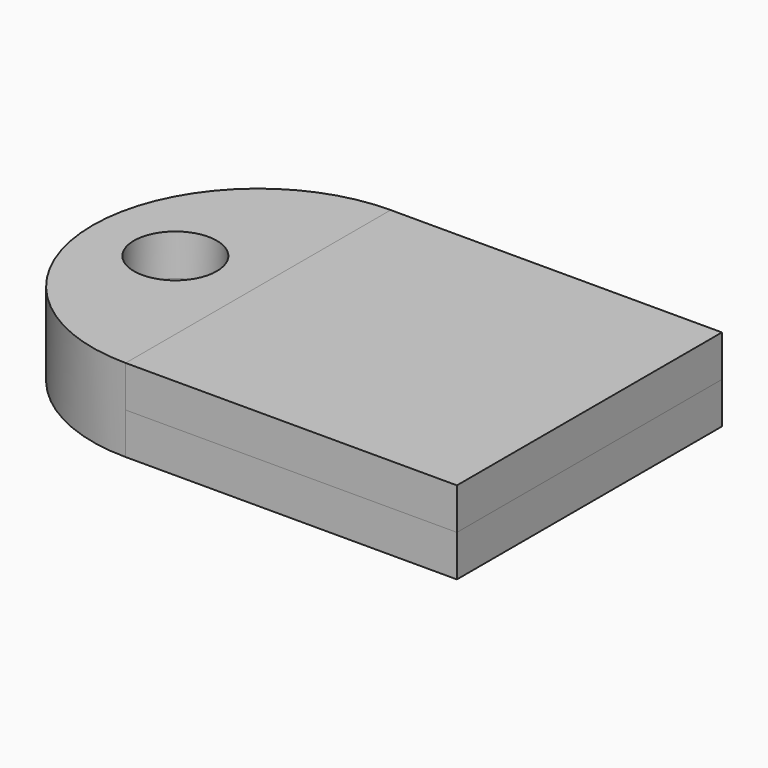
from build123d import *

# Parameters (mm, degrees)
F0_R          = 6.35
F1_DEPTH      = 6.35
F1_DEPTH_BACK = 6.35
F0_W          = 50.8
F0_H          = 50.8
F2_DEPTH      = 6.35
F3_DEPTH      = 6.35
F4_DEPTH      = 6.35


with BuildPart() as f1:
    # F0 (on Top) → F1 (new body, two sides)
    with BuildSketch(Plane.XY) as f1_sk:
        with BuildLine():
            Line((-25.4, -25.4), (-25.4, 25.4))
            ThreePointArc((-25.4, 25.4), (-50.8, 0), (-25.4, -25.4))
        make_face()
        with Locations((-38.1, 0)):
            Circle(F0_R, mode=Mode.SUBTRACT)
    extrude(amount=F1_DEPTH)
    extrude(f1_sk.sketch, amount=-F1_DEPTH_BACK)

    # F0 (on Top) → F2 (join)
    with BuildSketch(Plane.XY):
        Rectangle(F0_W, F0_H)
        with Locations((-12.7, -12.7)):
            Circle(F0_R, mode=Mode.SUBTRACT)
        with Locations((12.7, -12.7)):
            Circle(F0_R, mode=Mode.SUBTRACT)
        with Locations((-12.7, 12.7)):
            Circle(F0_R, mode=Mode.SUBTRACT)
        with Locations((12.7, 12.7)):
            Circle(F0_R, mode=Mode.SUBTRACT)
    extrude(amount=-F2_DEPTH)


with BuildPart() as f3:
    # F0 (on Top) → F3 (new body)
    with BuildSketch(Plane.XY):
        Rectangle(F0_W, F0_H)
        with Locations((-12.7, -12.7)):
            Circle(F0_R, mode=Mode.SUBTRACT)
        with Locations((12.7, -12.7)):
            Circle(F0_R, mode=Mode.SUBTRACT)
        with Locations((-12.7, 12.7)):
            Circle(F0_R, mode=Mode.SUBTRACT)
        with Locations((12.7, 12.7)):
            Circle(F0_R, mode=Mode.SUBTRACT)
        with Locations((-12.7, -12.7)):
            Circle(F0_R)
        with Locations((12.7, -12.7)):
            Circle(F0_R)
        with Locations((12.7, 12.7)):
            Circle(F0_R)
        with Locations((-12.7, 12.7)):
            Circle(F0_R)
    extrude(amount=F3_DEPTH)

    # F0 (on Top) → F4 (join)
    with BuildSketch(Plane.XY):
        with Locations((12.7, -12.7)):
            Circle(F0_R)
        with Locations((12.7, 12.7)):
            Circle(F0_R)
        with Locations((-12.7, 12.7)):
            Circle(F0_R)
        with Locations((-12.7, -12.7)):
            Circle(F0_R)
    extrude(amount=-F4_DEPTH)


solid = Compound([f1.part, f3.part])
